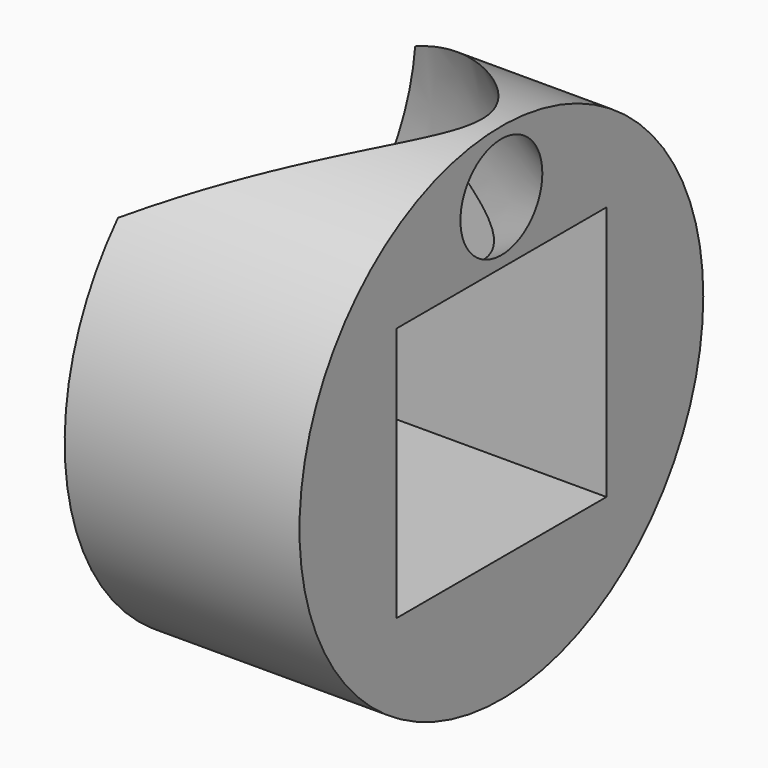
from build123d import *

# Parameters (mm, degrees)
F1_DEPTH = 67.31
F3_DEPTH = 91.186
F4_R     = 145.3123956035
F5_DEPTH = 135.2049764246
F6_W     = 151.2885987759
F6_H     = 146.8262225389
F7_DEPTH = 219.4037679583
F8_R     = 29.4822475013
F9_DEPTH = 135.2059764246
F9_TAPER = -30


# Not quite as in the source:
# - a feature of the source that left no trace in its solid (it failed there, or was rolled back) is left out


with BuildPart() as f1:
    # F0 (on Top) → F1 (new body)
    with BuildSketch(Plane.XY):
        Polygon((45.1956306257, 12.500264471), (26.5868465743, 38.6269495137), (-4.4622184691, 46.6796555882), (-33.4233618988, 32.8904320264), (-46.7453428367, 3.711409783), (-38.1946583448, -27.2042223456), (-11.7722687269, -45.3906964974), (20.1584962624, -42.3383592967), (42.6568768139, -19.4754332426), align=None)
    extrude(amount=F1_DEPTH)

    # F2 (on face) → F3 (cut)
    with BuildSketch(Plane.XY.offset(67.31)):
        Polygon((13.3602926508, -6.4339778404), (13.3602926508, 6.4339778404), (3.2997197844, 14.4570169783), (-9.2456093816, 11.593627462), (-14.8288061072, 0), (-9.2456093816, -11.593627462), (3.2997197844, -14.4570169783), align=None)
    extrude(amount=-F3_DEPTH, mode=Mode.SUBTRACT)

    # F4 (on Right) → F5 (join)
    with BuildSketch(Plane.YZ):
        Circle(F4_R)
    extrude(amount=F5_DEPTH)

    # F6 (on face) → F7 (cut)
    with BuildSketch(Plane.YZ.offset(135.2049764246)):
        Rectangle(F6_W, F6_H)
    extrude(amount=-F7_DEPTH, mode=Mode.SUBTRACT)

    # F8 (on face) → F9 (cut, through all)
    with BuildSketch(Plane.YZ.offset(135.2049764246)):
        with Locations((0, 109.3934327364)):
            Circle(F8_R)
    extrude(amount=-F9_DEPTH, taper=F9_TAPER, mode=Mode.SUBTRACT)


solid = f1.part
